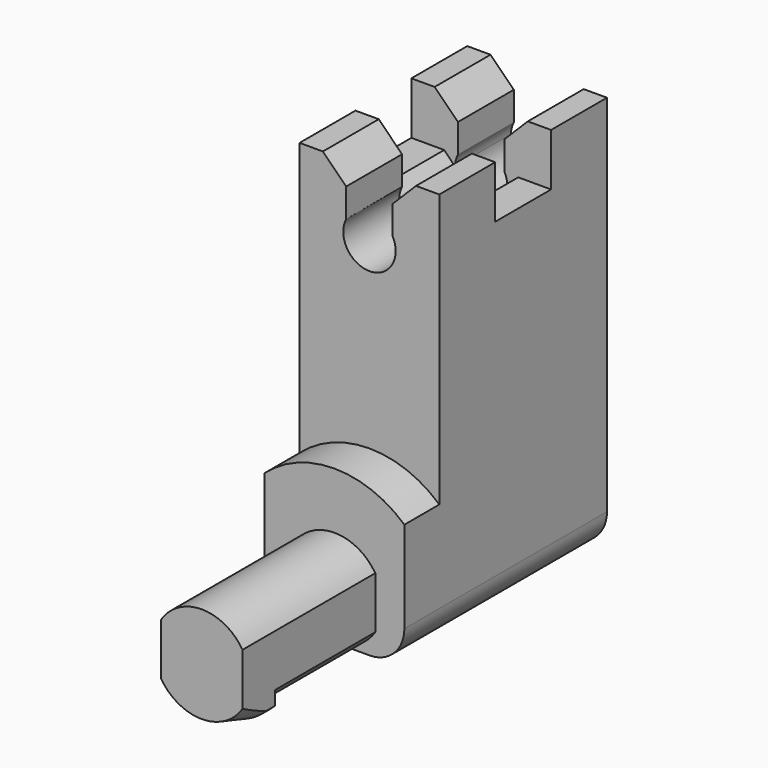
from build123d import *

# Parameters (mm, degrees)
F0_W         = 6
F0_H         = 18
F1_DEPTH     = 8
F3_DEPTH     = 18
F4_DEPTH     = 6
F5_DEPTH     = 4.2
F10_DEPTH    = 6
F11_R        = 2.25
F13_DEPTH    = 25
F14_W        = 4
F14_H        = 4.5
F15_DEPTH    = 25
F16_W        = 2.5
F16_H        = 17.5837995484
F16_W_2      = 3.5
F17_DEPTH    = 18.001
F18_W        = 2
F18_H        = 6
F19_DEPTH    = 30
F21_DEPTH    = 6
F23_DEPTH    = 3.75
F24_R        = 3
F26_DEPTH    = 25
F27_DEPTH    = 2
F28_T1_DEPTH = 16.2867319519
F30_DEPTH    = 6
F31_T1_DEPTH = 9.0166310888
F33_DEPTH    = 6


# Not quite as in the source:
# - a fillet or chamfer that OpenCascade refuses, or shapes differently, is made with other operations: its cross-section is extruded or revolved along the edge and cut away or added


with BuildPart() as f1:
    # F0 (on Right) → F1 (new body)
    with BuildSketch(Plane.YZ):
        with Locations((-22.1395939865, -6.3859075308)):
            Rectangle(F0_W, F0_H)
    extrude(amount=F1_DEPTH)


with BuildPart() as f3:
    # F2 (on face) → F3 (new body)
    with BuildSketch(Plane.XZ.offset(25.1395939865)):
        with BuildLine():
            ThreePointArc((4, -15.3859075308), (1.0655068581, -22.4704006727), (8.15, -19.5359075308))
            ThreePointArc((8.15, -19.5359075308), (6.9344931419, -16.6014143889), (4, -15.3859075308))
        make_face()
    extrude(amount=F3_DEPTH)


with BuildPart() as f4:
    # F4 (new, through all): a face of the model
    f4_faces = [f3.part.faces().sort_by_distance(p)[0] for p in [
        (4, -25.1395939865, -19.5359075308),
    ]]
    extrude(f4_faces, amount=F4_DEPTH)


with BuildPart() as f5:
    # F5 (new): a face of the model
    f5_faces = [f1.part.faces().sort_by_distance(p)[0] for p in [
        (4, -22.1395939865, -15.3859075308),
    ]]
    extrude(f5_faces, amount=F5_DEPTH)


with BuildPart() as f3_1:
    add(f3.part)

    # F6: union F4, F5, F1
    add(f4.part)
    add(f5.part)
    add(f1.part)

    # F8 (on mid) → F9 (revolve)
    with BuildSketch(Plane.YZ.offset(4)):
        Polygon((-43.1395939865, -15.3859075308), (-39.6395939865, -15.3859075308), (-39.6395939865, -14.6359075308), (-40.6395939865, -14.6359075308), align=None)
    revolve(axis=Axis((4, -25.1395939865, -19.5359075308), (0, 1, 0)))


with BuildPart() as f10:
    # F10 (new): a face of the model
    f10_faces = [f3_1.part.faces().sort_by_distance(p)[0] for p in [
        (4, -22.1395939865, 2.6140924692),
    ]]
    extrude(f10_faces, amount=F10_DEPTH)

    # F12: union F3
    add(f3_1.part)

    # F11 (on face) → F13 (cut)
    with BuildSketch(Plane(origin=(0, -19.1395939865, 0), x_dir=(-1, 0, 0), z_dir=(0, 1, 0))):
        with Locations((-4, 5.1140924692)):
            Circle(F11_R)
    extrude(amount=-F13_DEPTH, mode=Mode.SUBTRACT)

    # F14 (on face) → F15 (cut)
    with BuildSketch(Plane(origin=(0, -19.1395939865, 0), x_dir=(-1, 0, 0), z_dir=(0, 1, 0))):
        with Locations((-4, 7.3640924692)):
            Rectangle(F14_W, F14_H)
    extrude(amount=-F15_DEPTH, mode=Mode.SUBTRACT)

    # F16 (on face) → F17 (cut, through all)
    with BuildSketch(Plane.XZ.offset(25.1395939865)):
        with Locations((-0.75, -18.0519367568)):
            Rectangle(F16_W, F16_H)
        with Locations((9.25, -18.0519367568)):
            Rectangle(F16_W_2, F16_H)
    extrude(amount=F17_DEPTH, mode=Mode.SUBTRACT)

    # F18 (on face) → F19 (join)
    with BuildSketch(Plane.XY.offset(8.6140924692)):
        with Locations((-1, -22.1395939865)):
            Rectangle(F18_W, F18_H)
        with Locations((9, -22.1395939865)):
            Rectangle(F18_W, F18_H)
    extrude(amount=-F19_DEPTH)

    # F20 (on face) → F21 (join, through all)
    with BuildSketch(Plane(origin=(0, -19.1395939865, 0), x_dir=(-1, 0, 0), z_dir=(0, 1, 0))):
        with BuildLine():
            Line((-8, -21.3859075308), (-10, -21.3859075308))
            Line((-10, -21.3859075308), (-10, -23.6859075308))
            Line((-10, -23.6859075308), (-4, -23.6859075308))
            ThreePointArc((-4, -23.6859075308), (-6.5133623932, -22.8382566159), (-8, -20.6415747502))
            Line((-8, -20.6415747502), (-8, -21.3859075308))
        make_face()
        with BuildLine():
            Line((2, -23.6859075308), (2, -21.3859075308))
            Line((2, -21.3859075308), (0, -21.3859075308))
            Line((0, -21.3859075308), (0, -20.6415747502))
            ThreePointArc((0, -20.6415747502), (-1.4866376068, -22.8382566159), (-4, -23.6859075308))
            Line((-4, -23.6859075308), (2, -23.6859075308))
        make_face()
        with BuildLine():
            Line((2, -13.6859075308), (-10, -13.6859075308))
            Line((-10, -13.6859075308), (-10, -21.3859075308))
            Line((-10, -21.3859075308), (-8, -21.3859075308))
            Line((-8, -21.3859075308), (-8, -20.6415747502))
            ThreePointArc((-8, -20.6415747502), (-6.5133623932, -22.8382566159), (-4, -23.6859075308))
            ThreePointArc((-4, -23.6859075308), (-1.4866376068, -22.8382566159), (0, -20.6415747502))
            Line((0, -20.6415747502), (0, -21.3859075308))
            Line((0, -21.3859075308), (2, -21.3859075308))
            Line((2, -21.3859075308), (2, -13.6859075308))
        make_face()
    extrude(amount=-F21_DEPTH)

    # F22 (on face) → F23 (join)
    with BuildSketch(Plane.XZ.offset(25.1395939865)):
        with BuildLine():
            Line((10, -23.6859075308), (10, -12.8277035983))
            ThreePointArc((10, -12.8277035983), (4, -10.5359075308), (-2, -12.8277035983))
            Line((-2, -12.8277035983), (-2, -23.6859075308))
            Line((-2, -23.6859075308), (10, -23.6859075308))
        make_face()
    extrude(amount=F23_DEPTH)

    # F24
    f24_edges = [f10.edges().sort_by_distance(p)[0] for p in [
        (-2, -24.014594, -23.685908),
        (10, -24.014594, -23.685908),
    ]]
    fillet(f24_edges, radius=F24_R)

    # F25 (on face) → F26 (cut)
    with BuildSketch(Plane.XZ.offset(28.8895939865)):
        with BuildLine():
            ThreePointArc((-0.15, -19.5359075308), (4, -15.3859075308), (8.15, -19.5359075308))
            Line((8.15, -19.5359075308), (10, -19.5359075308))
            Line((10, -19.5359075308), (10, -10.5359075308))
            Line((10, -10.5359075308), (-2, -10.5359075308))
            Line((-2, -10.5359075308), (-2, -19.5359075308))
            Line((-2, -19.5359075308), (-0.15, -19.5359075308))
        make_face()
    extrude(amount=F26_DEPTH, mode=Mode.SUBTRACT)

    # F27 (add): faces of the model
    f27_faces = [f10.faces().sort_by_distance(p)[0] for p in [
        (0, -22.1395939865, 8.6140924692),
        (8, -22.1395939865, 8.6140924692),
    ]]
    extrude(f27_faces, amount=F27_DEPTH)

    # F28: chamfer of 2 on 4 edges, made by hand

    # F28_s2 → F28_t1 (cut)
    with BuildSketch(Plane.XZ.offset(13.9962280105)):
        Polygon((8, 10.6140924692), (6, 8.6140924692), (6, 10.6140924692), align=None)
        Polygon((2, 8.6140924692), (0, 10.6140924692), (2, 10.6140924692), align=None)
    extrude(amount=F28_T1_DEPTH, mode=Mode.SUBTRACT)

    # F29 (on face) → F30 (join)
    with BuildSketch(Plane(origin=(0, -19.1395939865, 0), x_dir=(-1, 0, 0), z_dir=(0, 1, 0))):
        with BuildLine():
            Line((-6.0155644371, 6.1140924692), (-10, 6.1140924692))
            Line((-10, 6.1140924692), (-10, -20.6859075308))
            ThreePointArc((-10, -20.6859075308), (-9.1213203436, -22.8072278743), (-7, -23.6859075308))
            Line((-7, -23.6859075308), (-1, -23.6859075308))
            ThreePointArc((-1, -23.6859075308), (1.1213203436, -22.8072278743), (2, -20.6859075308))
            Line((2, -20.6859075308), (2, 6.1140924692))
            Line((2, 6.1140924692), (-1.9844355629, 6.1140924692))
            ThreePointArc((-1.9844355629, 6.1140924692), (-4, 2.8640924692), (-6.0155644371, 6.1140924692))
        make_face()
    extrude(amount=F30_DEPTH)

    # F31: chamfer of 1.5 on 2 edges, made by hand

    # F31_s2 → F31_t1 (cut)
    with BuildSketch(Plane.XZ.offset(10.1229628977)):
        with BuildLine():
            Line((7.2214544106, 6.1569815348), (6.2075003037, 5.1205433408))
            Line((6.2075003037, 5.1205433408), (6.1775075177, 5.119885475))
            ThreePointArc((6.1775075177, 5.119885475), (6.1595192188, 5.6287542453), (5.9886902446, 6.1007591359))
            Line((5.9886902446, 6.1007591359), (6.0155644371, 6.1440924692))
            ThreePointArc((6.0155644371, 6.1440924692), (6.6185094238, 6.1440924692), (7.2214544106, 6.1869815348))
            Line((7.2214544106, 6.1869815348), (7.2214544106, 6.1569815348))
        make_face()
        with BuildLine():
            Line((0.7785455894, 6.1569815348), (1.7924996963, 5.1205433408))
            Line((1.7924996963, 5.1205433408), (1.8224924823, 5.119885475))
            ThreePointArc((1.8224924823, 5.119885475), (1.8404807812, 5.6287542453), (2.0113097554, 6.1007591359))
            Line((2.0113097554, 6.1007591359), (1.9844355629, 6.1440924692))
            ThreePointArc((1.9844355629, 6.1440924692), (1.3814905762, 6.1440924692), (0.7785455894, 6.1869815348))
            Line((0.7785455894, 6.1869815348), (0.7785455894, 6.1569815348))
        make_face()
    extrude(amount=F31_T1_DEPTH, mode=Mode.SUBTRACT)

    # F32 (on face) → F33 (join)
    with BuildSketch(Plane(origin=(0, -13.1395939865, 0), x_dir=(-1, 0, 0), z_dir=(0, 1, 0))):
        with BuildLine():
            ThreePointArc((-2, 6.1448688756), (-1.8193396117, 5.668367014), (-1.7505410494, 5.1634324064))
            Line((-1.7505410494, 5.1634324064), (-0.8205042363, 6.1140924692))
            Line((-0.8205042363, 6.1140924692), (2, 6.1140924692))
            Line((2, 6.1140924692), (2, 10.6140924692))
            Line((2, 10.6140924692), (0, 10.6140924692))
            Line((0, 10.6140924692), (-2, 8.6140924692))
            Line((-2, 8.6140924692), (-2, 6.1448688756))
        make_face()
        with BuildLine():
            Line((-8, 10.6140924692), (-10, 10.6140924692))
            Line((-10, 10.6140924692), (-10, 6.1140924692))
            Line((-10, 6.1140924692), (-7.1794957637, 6.1140924692))
            Line((-7.1794957637, 6.1140924692), (-6.2494589506, 5.1634324064))
            ThreePointArc((-6.2494589506, 5.1634324064), (-6.1806603883, 5.668367014), (-6, 6.1448688756))
            Line((-6, 6.1448688756), (-6, 8.6140924692))
            Line((-6, 8.6140924692), (-8, 10.6140924692))
        make_face()
        with BuildLine():
            Line((-7.1794957637, 6.1140924692), (-10, 6.1140924692))
            Line((-10, 6.1140924692), (-10, -12.8277035983))
            Line((-10, -12.8277035983), (-10, -20.6859075308))
            ThreePointArc((-10, -20.6859075308), (-9.1213203436, -22.8072278743), (-7, -23.6859075308))
            Line((-7, -23.6859075308), (-1, -23.6859075308))
            ThreePointArc((-1, -23.6859075308), (1.1213203436, -22.8072278743), (2, -20.6859075308))
            Line((2, -20.6859075308), (2, -12.8277035983))
            Line((2, -12.8277035983), (2, 6.1140924692))
            Line((2, 6.1140924692), (-0.8205042363, 6.1140924692))
            Line((-0.8205042363, 6.1140924692), (-1.7505410494, 5.1634324064))
            ThreePointArc((-1.7505410494, 5.1634324064), (-4, 2.8640924692), (-6.2494589506, 5.1634324064))
            Line((-6.2494589506, 5.1634324064), (-7.1794957637, 6.1140924692))
        make_face()
    extrude(amount=F33_DEPTH)


solid = f10.part
